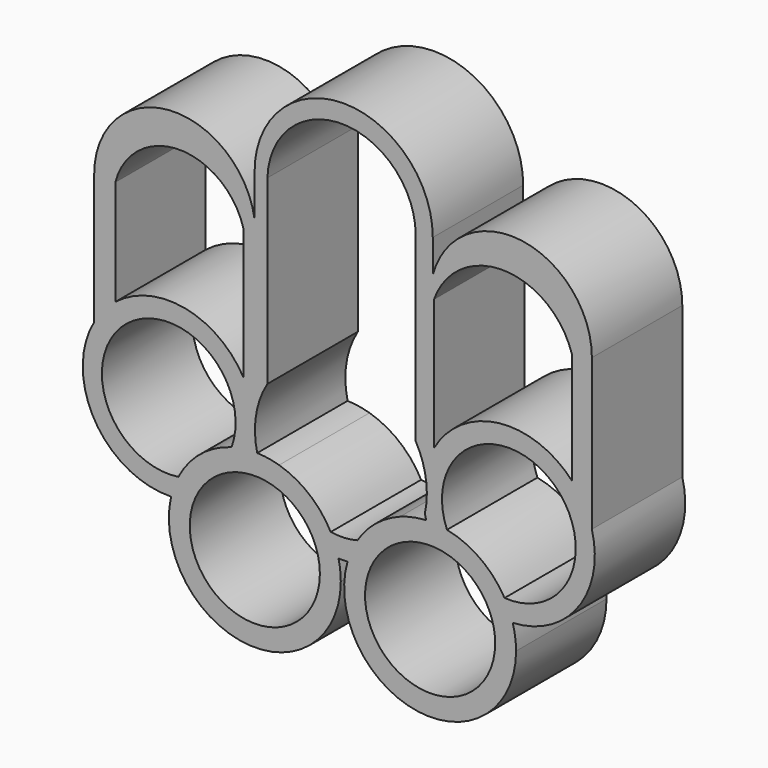
from build123d import *

# Parameters (mm, degrees)
F1_DEPTH = 30


# Not quite as in the source:
# - a feature of the source that left no trace in its solid (it failed there, or was rolled back) is left out
# - a feature names something its author has since deleted; it is built from what else it names


with BuildPart() as f1:
    # F0 (on Front) → F1 (new body)
    with BuildSketch(Plane.XZ):
        with BuildLine():
            ThreePointArc((-50.5958115044, -6.02955559), (-47.8576962726, -5.4409727065), (-45.0680997666, -5.1922637066))
            ThreePointArc((-45.0680997666, -5.1922637066), (-44.7014233398, 3.2450721847), (-47.4287139254, 11.2378798646))
            ThreePointArc((-47.4287139254, 11.2378798646), (-62.9262479802, 22.3973362627), (-81.478701042, 17.868151538))
            ThreePointArc((-81.478701042, 17.868151538), (-84.5846312596, 14.8818765302), (-87.0738165711, 11.3649748506))
            ThreePointArc((-87.0738165711, 11.3649748506), (-86.8766386462, -11.7015650942), (-66.6597911749, -22.8093651683))
            ThreePointArc((-66.6597911749, -22.8093651683), (-65.8563320665, -20.1264267988), (-64.7302441516, -17.5621275103))
            ThreePointArc((-64.7302441516, -17.5621275103), (-78.5071405294, 13.7509063134), (-50.5958115044, -6.02955559))
        make_face()
        with BuildLine():
            ThreePointArc((-47.4287139254, 11.2378798646), (-44.7014233398, 3.2450721847), (-45.0680997666, -5.1922637066))
            ThreePointArc((-45.0680997666, -5.1922637066), (-44.4403953733, -5.1836282573), (-43.8126909801, -5.1922637066))
            ThreePointArc((-43.8126909801, -5.1922637066), (-44.1262374484, 3.5955062023), (-41.0934242922, 11.8493087029))
            Line((-41.0934242922, 11.8493087029), (-41.0934242922, 59.9904626227))
            ThreePointArc((-41.0934242922, 59.9904626227), (-21.1129667901, 79.0608636102), (-1.7345135358, 59.3790337844))
            Line((-1.7345135358, 59.3790337844), (-1.7345135358, 11.2378798646))
            ThreePointArc((-1.7345135358, 11.2378798646), (-0.2806344187, 8.1505609331), (0.6965577317, 4.8809434977))
            ThreePointArc((0.6965577317, 4.8809434977), (1.6737498821, 8.1505609331), (3.1276289991, 11.2378798646))
            Line((3.1276289991, 11.2378798646), (3.1276289991, 45.9835585246))
            ThreePointArc((3.1276289991, 45.9835585246), (21.7197442499, 58.7768351813), (39.7009037986, 45.1381923457))
            Line((39.7009037986, 45.1381923457), (39.7009037986, 15.5334114315))
            ThreePointArc((39.7009037986, 15.5334114315), (42.9557629485, 11.0402047373), (45.0299754174, 5.8942687567))
            Line((45.0299754174, 5.8942687567), (45.0299754174, 45.9835585246))
            ThreePointArc((45.0299754174, 45.9835585246), (26.3569721709, 67.2830168196), (2.7973072292, 51.5575546089))
            Line((2.7973072292, 51.5575546089), (2.7973072292, 60.3419492483))
            ThreePointArc((2.7973072292, 60.3419492483), (-21.0300426798, 83.9928980167), (-44.5032843921, 59.9904626227))
            Line((-44.5032843921, 59.9904626227), (-44.5032843921, 49.1925225526))
            ThreePointArc((-44.5032843921, 49.1925225526), (-67.2766387272, 67.32921183), (-87.0738165711, 45.9835585246))
            Line((-87.0738165711, 45.9835585246), (-87.0738165711, 11.3649748506))
            ThreePointArc((-87.0738165711, 11.3649748506), (-84.5846312596, 14.8818765302), (-81.478701042, 17.868151538))
            Line((-81.478701042, 17.868151538), (-81.478701042, 45.8139192271))
            ThreePointArc((-81.478701042, 45.8139192271), (-64.5188702281, 58.9782000656), (-47.4287139254, 45.9835585246))
            Line((-47.4287139254, 45.9835585246), (-47.4287139254, 11.2378798646))
        make_face()
        with BuildLine():
            ThreePointArc((-43.8126909801, -5.1922637066), (-44.4403953733, -5.1836282573), (-45.0680997666, -5.1922637066))
            ThreePointArc((-45.0680997666, -5.1922637066), (-47.8576962726, -5.4409727065), (-50.5958115044, -6.02955559))
            ThreePointArc((-50.5958115044, -6.02955559), (-58.8656531806, -10.3218921863), (-64.7302441516, -17.5621275103))
            ThreePointArc((-64.7302441516, -17.5621275103), (-65.8563320665, -20.1264267988), (-66.6597911749, -22.8093651683))
            ThreePointArc((-66.6597911749, -22.8093651683), (-47.0537232386, -50.6694843019), (-21.6223947557, -28.001628875))
            ThreePointArc((-21.6223947557, -28.001628875), (-21.7725399464, -25.3883010097), (-22.2209995718, -22.8093651683))
            ThreePointArc((-22.2209995718, -22.8093651683), (-23.0778257417, -19.9827903731), (-24.2925817064, -17.2905711947))
            ThreePointArc((-24.2925817064, -17.2905711947), (-30.0151375661, -10.3218921863), (-37.9904438403, -6.1142060617))
            ThreePointArc((-37.9904438403, -6.1142060617), (-40.8716704219, -5.4644295279), (-43.8126909801, -5.1922637066))
        make_face()
        with BuildLine():
            ThreePointArc((-28.3212575169, -21.8035702343), (-27.4607721402, -24.8496563168), (-27.1706954296, -28.001628875))
            ThreePointArc((-27.1706954296, -28.001628875), (-47.5923679315, -44.9812521081), (-60.5595332298, -21.8035702343))
            ThreePointArc((-60.5595332298, -21.8035702343), (-55.3580861087, -14.6208006063), (-47.2776192349, -10.9665856726))
            ThreePointArc((-47.2776192349, -10.9665856726), (-44.4403953733, -10.7319289312), (-41.6031715118, -10.9665856726))
            ThreePointArc((-41.6031715118, -10.9665856726), (-33.522704638, -14.6208006063), (-28.3212575169, -21.8035702343))
        make_face(mode=Mode.SUBTRACT)
        with BuildLine():
            ThreePointArc((-17.209328187, -16.9419843412), (-20.7331119046, -17.4788467793), (-24.2925817064, -17.2905711947))
            ThreePointArc((-24.2925817064, -17.2905711947), (-23.0778257417, -19.9827903731), (-22.2209995718, -22.8093651683))
            ThreePointArc((-22.2209995718, -22.8093651683), (-21.0207224268, -22.8108156941), (-19.8220295884, -22.749148784))
            ThreePointArc((-19.8220295884, -22.749148784), (-18.7192509321, -19.7539774624), (-17.209328187, -16.9419843412))
        make_face()
        with BuildLine():
            ThreePointArc((0.318409666, -6.3669728281), (-2.8385741788, -6.8366801987), (-5.8991326911, -7.7423035215))
            ThreePointArc((-5.8991326911, -7.7423035215), (-12.3087515473, -11.4145268316), (-17.209328187, -16.9419843412))
            ThreePointArc((-17.209328187, -16.9419843412), (-18.7192509321, -19.7539774624), (-19.8220295884, -22.749148784))
            ThreePointArc((-19.8220295884, -22.749148784), (-1.125900704, -51.7064120801), (24.9076758738, -29.1161216121))
            ThreePointArc((24.9076758738, -29.1161216121), (24.6833038658, -25.92408489), (24.0146003931, -22.7948234918))
            ThreePointArc((24.0146003931, -22.7948234918), (23.0881839229, -20.1873038876), (21.8529406759, -17.7111011327))
            ThreePointArc((21.8529406759, -17.7111011327), (15.3942852462, -10.5783627076), (6.5696450929, -6.7422300764))
            ThreePointArc((6.5696450929, -6.7422300764), (3.8283507197, -6.3644588197), (1.0614855049, -6.3212981203))
            ThreePointArc((1.0614855049, -6.3212981203), (0.6897612956, -6.3411047495), (0.318409666, -6.3669728281))
        make_face()
        with BuildLine():
            ThreePointArc((19.3593751999, -29.1161216121), (-10.6177327064, -40.8107493967), (3.5207306993, -11.9058160812))
            ThreePointArc((3.5207306993, -11.9058160812), (12.1592087901, -15.0859031335), (17.936744923, -22.2522364789))
            ThreePointArc((17.936744923, -22.2522364789), (18.9999779483, -25.6112394448), (19.3593751999, -29.1161216121))
        make_face(mode=Mode.SUBTRACT)
        with BuildLine():
            ThreePointArc((3.1276289991, 11.2378798646), (1.6737498821, 8.1505609331), (0.6965577317, 4.8809434977))
            ThreePointArc((0.6965577317, 4.8809434977), (1.2247054391, 0), (0.6965577317, -4.8809434977))
            ThreePointArc((0.6965577317, -4.8809434977), (0.8672943666, -5.6040920216), (1.0614855049, -6.3212981203))
            ThreePointArc((1.0614855049, -6.3212981203), (3.8283507197, -6.3644588197), (6.5696450929, -6.7422300764))
            ThreePointArc((6.5696450929, -6.7422300764), (33.3344406342, 14.4182569257), (21.8529406759, -17.7111011327))
            ThreePointArc((21.8529406759, -17.7111011327), (23.0881839229, -20.1873038876), (24.0146003931, -22.7948234918))
            ThreePointArc((24.0146003931, -22.7948234918), (41.3940847955, -13.484015887), (45.0299754174, 5.8942687567))
            ThreePointArc((45.0299754174, 5.8942687567), (42.9557629485, 11.0402047373), (39.7009037986, 15.5334114315))
            ThreePointArc((39.7009037986, 15.5334114315), (20.3247315889, 22.6622288579), (3.1276289991, 11.2378798646))
        make_face()
    extrude(amount=F1_DEPTH)


solid = f1.part
